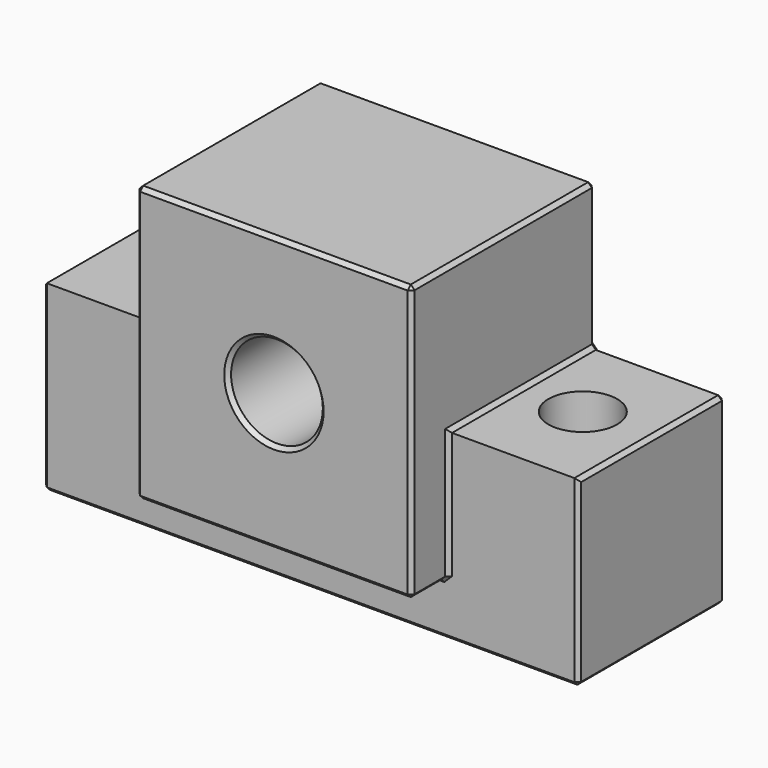
from build123d import *

# Parameters (mm, degrees)
F0_R     = 6
F1_DEPTH = 12
F2_R     = 6
F3_DEPTH = 6
F5_D     = 9
F6_SIZE  = 0.5


with BuildPart() as f1:
    # F0 (on Front) → F1 (new body, symmetric)
    with BuildSketch(Plane.XZ):
        Polygon((18, 18), (0, 18), (-18, 18), (-18, -1), (-35, -1), (-35, -25), (0, -25), (35, -25), (35, -1), (18, -1), align=None)
        Circle(F0_R, mode=Mode.SUBTRACT)
    extrude(amount=F1_DEPTH, both=True)

    # F2 (on face) → F3 (join)
    with BuildSketch(Plane.XZ.offset(12)):
        Polygon((18, 18), (-18, 18), (-18, -1), (-18, -18), (18, -18), (18, -1), align=None)
        Circle(F2_R, mode=Mode.SUBTRACT)
    extrude(amount=F3_DEPTH)

    # F5 (through all)
    with Locations(Plane(origin=(0, 0, -25), x_dir=(1, 0, 0), z_dir=(0, 0, -1))):
        with Locations((-26, 0), (26, 0)):
            Hole(F5_D / 2)

    # F6
    f6_edges = [f1.edges().sort_by_distance(p)[0] for p in [
        (18, -3, 18),
        (-18, -3, 18),
        (0, -18, 18),
        (-18, -18, 0),
        (0, -18, -18),
        (18, -18, 0),
        (-6, -18, 0),
        (35, 0, -25),
        (35, 12, -13),
        (35, 0, -1),
        (35, -12, -13),
        (26.5, 12, -1),
        (18, 12, 8.5),
        (0, 12, 18),
        (-26.5, 12, -1),
        (-18, 12, 8.5),
        (-18, 0, -1),
        (-18, -12, -9.5),
        (-18, -15, -18),
        (18, -15, -18),
        (18, -12, -9.5),
        (18, 0, -1),
        (0, 12, -25),
        (-35, 0, -1),
        (-35, 12, -13),
        (-35, 0, -25),
        (-35, -12, -13),
        (0, -12, -25),
        (0, -12, -18),
    ]]
    chamfer(f6_edges, length=F6_SIZE)


solid = f1.part
